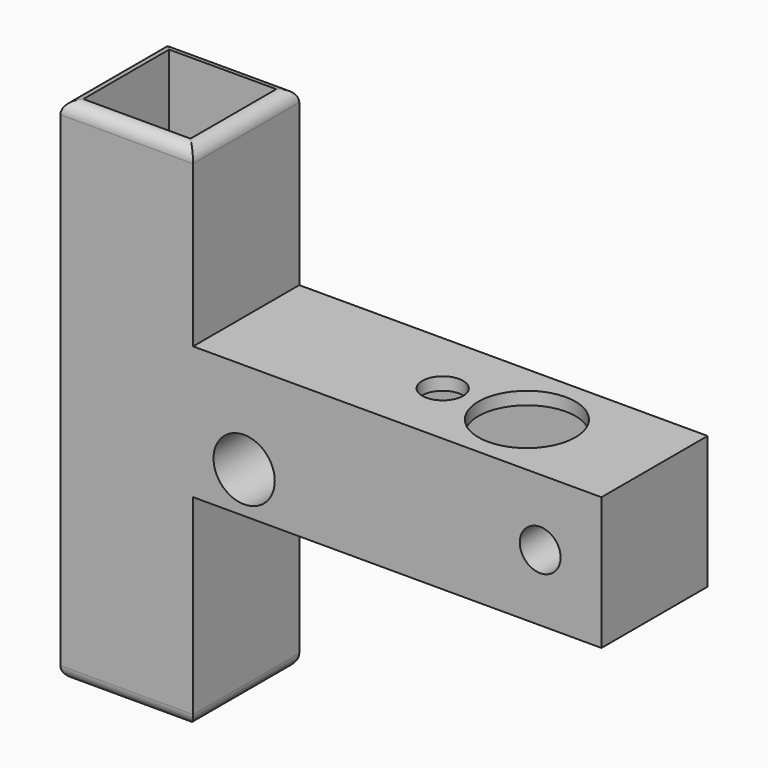
from build123d import *

# Parameters (mm, degrees)
F0_W        = 80
F0_H        = 26
F0_R        = 6
F0_R_2      = 4
F1_DEPTH    = 13
F2_T        = 2.5
F2_T3_DEPTH = 31
F3_R        = 9.5
F3_R_2      = 4
F4_DEPTH    = 50
F5_R        = 2.49999


# Not quite as in the source:
# - a fillet or chamfer is up to 0.001 mm smaller than in the source, because OpenCascade refuses the exact size
# - a shell that OpenCascade refuses in one call is made with other operations: the cavity is built on its own and cut out


with BuildPart() as f1:
    # F0 (on Front) → F1 (new body, symmetric)
    with BuildSketch(Plane.XZ):
        Polygon((0, 25.9917649148), (0, 59.9917649148), (-26, 59.9917649148), (-26, -40.0082350852), (0, -40.0082350852), (0, -0.0082350852), align=None)
        with Locations((40, 12.9917649148)):
            Rectangle(F0_W, F0_H)
        with Locations((10, 7.9917649148)):
            Circle(F0_R, mode=Mode.SUBTRACT)
        with Locations((68, 12.9917649148)):
            Circle(F0_R_2, mode=Mode.SUBTRACT)
    extrude(amount=F1_DEPTH, both=True)

    # F2: shell of thickness 2.5, made by hand


with BuildPart() as f2_core1:
    # F2_t2: copy of F1
    add(f1.part)

    # the walls: a layer under each face that stays
    f2_faces = [f2_core1.faces().sort_by_distance(p)[0] for p in [
        (0, 0, 42.9917649148),
        (40, 0, 25.9917649148),
        (80, 0, 12.9917649148),
        (40, 0, -0.0082350852),
        (0, 0, -20.0082350852),
        (-26, 0, 9.9917649148),
        (27, -13, 9.9917649148),
        (4, 0, 7.9917649148),
        (64, 0, 12.9917649148),
        (27, 13, 9.9917649148),
    ]]
    thicken(f2_faces, amount=-F2_T, mode=Mode.SUBTRACT)

    # F2_s4 → F2_t3 (cut)
    with BuildSketch(Plane.XZ.offset(-15.5)):
        Polygon((0.025, 26.0167649148), (-2.5, 25.9917649148), (-2.5, 23.4917649148), (0, 23.4917649148), align=None)
        Polygon((0.025, -0.0332350852), (0, 2.4917649148), (-2.5, 2.4917649148), (-2.5, -0.0082350852), align=None)
    extrude(amount=F2_T3_DEPTH, mode=Mode.SUBTRACT)


with BuildPart() as f1_1:
    add(f1.part)

    # what is left inside the walls is the cavity
    f2_cavity = [f2_core1.part.solids().sort_by_distance(p)[0] for p in [
        (-10.875, 10.475, 4.436209),
    ]]
    add(f2_cavity, mode=Mode.SUBTRACT)

    # F3 (on Top) → F4 (cut, symmetric)
    with BuildSketch(Plane.XY):
        with Locations((55, 0)):
            Circle(F3_R)
        with Locations((38.5, 0)):
            Circle(F3_R_2)
    extrude(amount=F4_DEPTH, both=True, mode=Mode.SUBTRACT)

    # F5 (radius 2.5 in the source; OpenCascade refuses exactly that, so slightly less here)
    f5_edges = [f1_1.edges().sort_by_distance(p)[0] for p in [
        (0, 0, 59.991765),
        (-13, -13, 59.991765),
        (-13, 13, 59.991765),
        (-26, 0, 59.991765),
        (-26, 0, -40.008235),
        (-13, 13, -40.008235),
        (0, 0, -40.008235),
        (-13, -13, -40.008235),
    ]]
    fillet(f5_edges, radius=F5_R)


solid = f1_1.part
